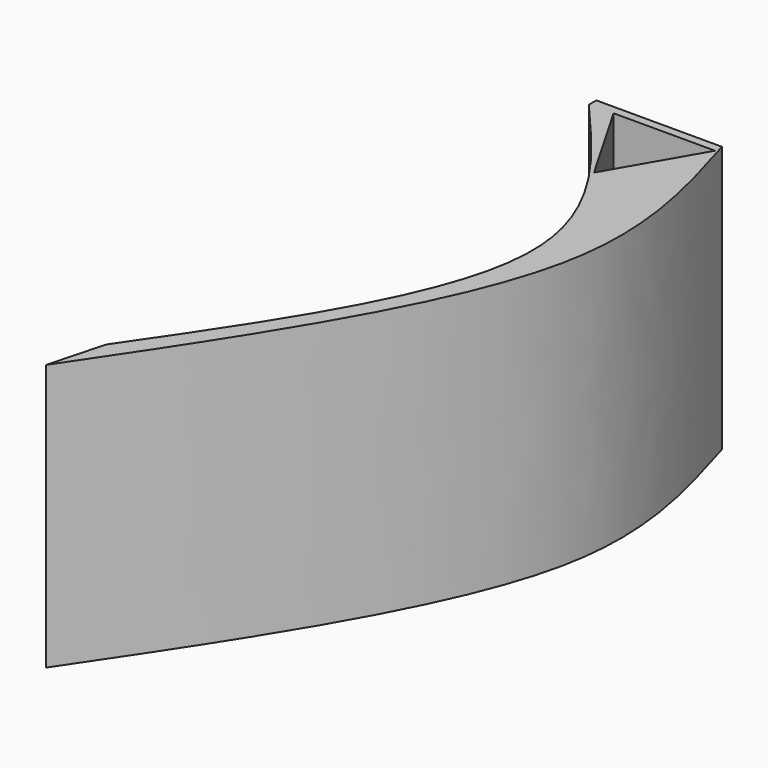
from build123d import *

# Parameters (mm, degrees)
F4_DEPTH = 102.616


# Not quite as in the source:
# - a feature of the source that left no trace in its solid (it failed there, or was rolled back) is left out


with BuildPart() as f4:
    # F3 (on Top) → F4 (new body)
    with BuildSketch(Plane.XY):
        with BuildLine():
            Line((-116.903886199, 40.9632176161), (-116.903886199, 37.3379997909))
            add(Edge.make_bspline(
                [(-116.903886199, 37.3379997909), (-94.3898521159, 11.5008250837), (-44.1040481936, -46.2073180434), (-101.1608146078, -129.3041537381), (-132.6720416546, -175.1967519522)],
                knots=[0, 0, 0, 0, 0.4477214706, 1, 1, 1, 1], degree=3))
            add(Edge.make_bspline(
                [(-138.4897381067, -196.8956440687), (-136.550505956, -189.6626800299), (-134.6112738053, -182.429715991), (-132.6720416546, -175.1967519522)],
                knots=[0, 0, 0, 0, 22.4652511914, 22.4652511914, 22.4652511914, 22.4652511914], degree=3))
            add(Edge.make_bspline(
                [(-68.5538262124, 40.9632176161), (-60.3988212358, 13.7210225854), (-40.7807645704, -51.8140601445), (-102.453603187, -143.3879738574), (-138.4897381067, -196.8956440687)],
                knots=[0, 0, 0, 0, 0.4156887257, 1, 1, 1, 1], degree=3))
            Line((-68.5538262124, 40.9632176161), (-116.903886199, 40.9632176161))
        make_face()
        Polygon((-88.0872011185, 3.8100015372), (-107.6205760246, 37.6427993178), (-68.5538262124, 37.6427993178), align=None, mode=Mode.SUBTRACT)
    extrude(amount=F4_DEPTH)


solid = f4.part
